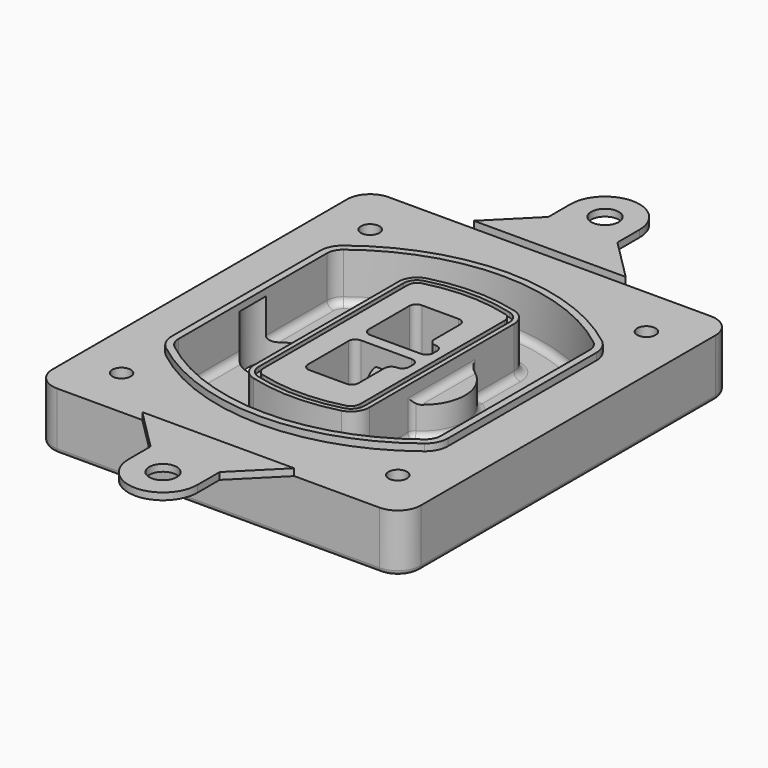
from build123d import *

# Parameters (mm, degrees)
F0_R      = 4
F1_DEPTH  = 25
F2_DEPTH  = 3
F3_DEPTH  = 18
F5_DEPTH  = 21
F6_DEPTH  = 2
F8_DEPTH  = 20
F9_DEPTH  = 16
F10_DEPTH = 25
F7_R      = 6
F7_R_2    = 4
F11_DEPTH = 6
F13_DEPTH = 9
F14_R     = 3
F15_R     = 2
F16_R     = 6
F17_DEPTH = 3


with BuildPart() as f1:
    # F0 (on Top) → F1 (new body)
    with BuildSketch(Plane.XY):
        with BuildLine():
            ThreePointArc((-80, -80), (-77.0710678119, -87.0710678119), (-70, -90))
            Line((-70, -90), (70, -90))
            ThreePointArc((70, -90), (77.0710678119, -87.0710678119), (80, -80))
            Line((80, -80), (80, 80))
            ThreePointArc((80, 80), (77.0710678119, 87.0710678119), (70, 90))
            Line((70, 90), (-70, 90))
            ThreePointArc((-70, 90), (-77.0710678119, 87.0710678119), (-80, 80))
            Line((-80, 80), (-80, -80))
        make_face()
        with Locations((-60, -67.5)):
            Circle(F0_R, mode=Mode.SUBTRACT)
        with Locations((60, -67.5)):
            Circle(F0_R, mode=Mode.SUBTRACT)
        with Locations((-60, 67.5)):
            Circle(F0_R, mode=Mode.SUBTRACT)
        with BuildLine():
            ThreePointArc((-64, 40.2934422872), (-62.5820384798, 46.4328484224), (-58.6153846154, 51.3286200352))
            ThreePointArc((-58.6153846154, 51.3286200352), (0, 71.5), (58.6153846154, 51.3286200352))
            ThreePointArc((58.6153846154, 51.3286200352), (62.5820384798, 46.4328484224), (64, 40.2934422872))
            Line((64, 40.2934422872), (64, -40.2934422872))
            ThreePointArc((64, -40.2934422872), (62.5820384798, -46.4328484224), (58.6153846154, -51.3286200352))
            ThreePointArc((58.6153846154, -51.3286200352), (0, -71.5), (-58.6153846154, -51.3286200352))
            ThreePointArc((-58.6153846154, -51.3286200352), (-62.5820384798, -46.4328484224), (-64, -40.2934422872))
            Line((-64, -40.2934422872), (-64, 40.2934422872))
        make_face(mode=Mode.SUBTRACT)
        with Locations((60, 67.5)):
            Circle(F0_R, mode=Mode.SUBTRACT)
        with BuildLine():
            ThreePointArc((58.6153846154, 51.3286200352), (0, 71.5), (-58.6153846154, 51.3286200352))
            ThreePointArc((-58.6153846154, 51.3286200352), (-62.5820384798, 46.4328484224), (-64, 40.2934422872))
            Line((-64, 40.2934422872), (-64, -40.2934422872))
            ThreePointArc((-64, -40.2934422872), (-62.5820384798, -46.4328484224), (-58.6153846154, -51.3286200352))
            ThreePointArc((-58.6153846154, -51.3286200352), (0, -71.5), (58.6153846154, -51.3286200352))
            ThreePointArc((58.6153846154, -51.3286200352), (62.5820384798, -46.4328484224), (64, -40.2934422872))
            Line((64, -40.2934422872), (64, 40.2934422872))
            ThreePointArc((64, 40.2934422872), (62.5820384798, 46.4328484224), (58.6153846154, 51.3286200352))
        make_face()
        with BuildLine():
            Line((-60, -40.2934422872), (-60, 40.2934422872))
            ThreePointArc((-60, 40.2934422872), (-58.9871703427, 44.6787323838), (-56.1538461538, 48.1757121072))
            ThreePointArc((-56.1538461538, 48.1757121072), (0, 67.5), (56.1538461538, 48.1757121072))
            ThreePointArc((56.1538461538, 48.1757121072), (58.9871703427, 44.6787323838), (60, 40.2934422872))
            Line((60, 40.2934422872), (60, -40.2934422872))
            ThreePointArc((60, -40.2934422872), (58.9871703427, -44.6787323838), (56.1538461538, -48.1757121072))
            ThreePointArc((56.1538461538, -48.1757121072), (0, -67.5), (-56.1538461538, -48.1757121072))
            ThreePointArc((-56.1538461538, -48.1757121072), (-58.9871703427, -44.6787323838), (-60, -40.2934422872))
        make_face(mode=Mode.SUBTRACT)
        with BuildLine():
            ThreePointArc((-56.1538461538, 48.1757121072), (-58.9871703427, 44.6787323838), (-60, 40.2934422872))
            Line((-60, 40.2934422872), (-60, -40.2934422872))
            ThreePointArc((-60, -40.2934422872), (-58.9871703427, -44.6787323838), (-56.1538461538, -48.1757121072))
            ThreePointArc((-56.1538461538, -48.1757121072), (0, -67.5), (56.1538461538, -48.1757121072))
            ThreePointArc((56.1538461538, -48.1757121072), (58.9871703427, -44.6787323838), (60, -40.2934422872))
            Line((60, -40.2934422872), (60, 40.2934422872))
            ThreePointArc((60, 40.2934422872), (58.9871703427, 44.6787323838), (56.1538461538, 48.1757121072))
            ThreePointArc((56.1538461538, 48.1757121072), (0, 67.5), (-56.1538461538, 48.1757121072))
        make_face()
        with BuildLine():
            ThreePointArc((54.3076923077, 45.8110311612), (56.2910192399, 43.3631453548), (57, 40.2934422872))
            Line((57, 40.2934422872), (57, -40.2934422872))
            ThreePointArc((57, -40.2934422872), (56.2910192399, -43.3631453548), (54.3076923077, -45.8110311612))
            ThreePointArc((54.3076923077, -45.8110311612), (0, -64.5), (-54.3076923077, -45.8110311612))
            ThreePointArc((-54.3076923077, -45.8110311612), (-56.2910192399, -43.3631453548), (-57, -40.2934422872))
            Line((-57, -40.2934422872), (-57, 40.2934422872))
            ThreePointArc((-57, 40.2934422872), (-56.2910192399, 43.3631453548), (-54.3076923077, 45.8110311612))
            ThreePointArc((-54.3076923077, 45.8110311612), (0, 64.5), (54.3076923077, 45.8110311612))
        make_face(mode=Mode.SUBTRACT)
        with BuildLine():
            Line((57, -40.2934422872), (57, 40.2934422872))
            ThreePointArc((57, 40.2934422872), (56.2910192399, 43.3631453548), (54.3076923077, 45.8110311612))
            ThreePointArc((54.3076923077, 45.8110311612), (0, 64.5), (-54.3076923077, 45.8110311612))
            ThreePointArc((-54.3076923077, 45.8110311612), (-56.2910192399, 43.3631453548), (-57, 40.2934422872))
            Line((-57, 40.2934422872), (-57, -40.2934422872))
            ThreePointArc((-57, -40.2934422872), (-56.2910192399, -43.3631453548), (-54.3076923077, -45.8110311612))
            ThreePointArc((-54.3076923077, -45.8110311612), (0, -64.5), (54.3076923077, -45.8110311612))
            ThreePointArc((54.3076923077, -45.8110311612), (56.2910192399, -43.3631453548), (57, -40.2934422872))
        make_face()
    extrude(amount=-F1_DEPTH)

    # F0 (on Top) → F2 (join)
    with BuildSketch(Plane.XY):
        with BuildLine():
            ThreePointArc((-56.1538461538, 48.1757121072), (-58.9871703427, 44.6787323838), (-60, 40.2934422872))
            Line((-60, 40.2934422872), (-60, -40.2934422872))
            ThreePointArc((-60, -40.2934422872), (-58.9871703427, -44.6787323838), (-56.1538461538, -48.1757121072))
            ThreePointArc((-56.1538461538, -48.1757121072), (0, -67.5), (56.1538461538, -48.1757121072))
            ThreePointArc((56.1538461538, -48.1757121072), (58.9871703427, -44.6787323838), (60, -40.2934422872))
            Line((60, -40.2934422872), (60, 40.2934422872))
            ThreePointArc((60, 40.2934422872), (58.9871703427, 44.6787323838), (56.1538461538, 48.1757121072))
            ThreePointArc((56.1538461538, 48.1757121072), (0, 67.5), (-56.1538461538, 48.1757121072))
        make_face()
        with BuildLine():
            ThreePointArc((54.3076923077, 45.8110311612), (56.2910192399, 43.3631453548), (57, 40.2934422872))
            Line((57, 40.2934422872), (57, -40.2934422872))
            ThreePointArc((57, -40.2934422872), (56.2910192399, -43.3631453548), (54.3076923077, -45.8110311612))
            ThreePointArc((54.3076923077, -45.8110311612), (0, -64.5), (-54.3076923077, -45.8110311612))
            ThreePointArc((-54.3076923077, -45.8110311612), (-56.2910192399, -43.3631453548), (-57, -40.2934422872))
            Line((-57, -40.2934422872), (-57, 40.2934422872))
            ThreePointArc((-57, 40.2934422872), (-56.2910192399, 43.3631453548), (-54.3076923077, 45.8110311612))
            ThreePointArc((-54.3076923077, 45.8110311612), (0, 64.5), (54.3076923077, 45.8110311612))
        make_face(mode=Mode.SUBTRACT)
    extrude(amount=F2_DEPTH)

    # F0 (on Top) → F3 (cut)
    with BuildSketch(Plane.XY):
        with BuildLine():
            Line((57, -40.2934422872), (57, 40.2934422872))
            ThreePointArc((57, 40.2934422872), (56.2910192399, 43.3631453548), (54.3076923077, 45.8110311612))
            ThreePointArc((54.3076923077, 45.8110311612), (0, 64.5), (-54.3076923077, 45.8110311612))
            ThreePointArc((-54.3076923077, 45.8110311612), (-56.2910192399, 43.3631453548), (-57, 40.2934422872))
            Line((-57, 40.2934422872), (-57, -40.2934422872))
            ThreePointArc((-57, -40.2934422872), (-56.2910192399, -43.3631453548), (-54.3076923077, -45.8110311612))
            ThreePointArc((-54.3076923077, -45.8110311612), (0, -64.5), (54.3076923077, -45.8110311612))
            ThreePointArc((54.3076923077, -45.8110311612), (56.2910192399, -43.3631453548), (57, -40.2934422872))
        make_face()
    extrude(amount=-F3_DEPTH, mode=Mode.SUBTRACT)

    # F4 (on face) → F5 (join, through all)
    with BuildSketch(Plane.XY.offset(3)):
        with BuildLine():
            ThreePointArc((-25, -39.2465276821), (-23.3511545998, -44.1109737193), (-19.0842911877, -46.9702398883))
            ThreePointArc((-19.0842911877, -46.9702398883), (0, -49.5), (19.0842911877, -46.9702398883))
            ThreePointArc((19.0842911877, -46.9702398883), (23.3511545998, -44.1109737193), (25, -39.2465276821))
            Line((25, -39.2465276821), (25, 39.2465276821))
            ThreePointArc((25, 39.2465276821), (23.3511545998, 44.1109737193), (19.0842911877, 46.9702398883))
            ThreePointArc((19.0842911877, 46.9702398883), (0, 49.5), (-19.0842911877, 46.9702398883))
            ThreePointArc((-19.0842911877, 46.9702398883), (-23.3511545998, 44.1109737193), (-25, 39.2465276821))
            Line((-25, 39.2465276821), (-25, -39.2465276821))
        make_face()
        with BuildLine():
            ThreePointArc((18.5632183908, 45.0393118368), (21.7633659499, 42.89486221), (23, 39.2465276821))
            Line((23, 39.2465276821), (23, -39.2465276821))
            ThreePointArc((23, -39.2465276821), (21.7633659499, -42.89486221), (18.5632183908, -45.0393118368))
            ThreePointArc((18.5632183908, -45.0393118368), (0, -47.5), (-18.5632183908, -45.0393118368))
            ThreePointArc((-18.5632183908, -45.0393118368), (-21.7633659499, -42.89486221), (-23, -39.2465276821))
            Line((-23, -39.2465276821), (-23, 39.2465276821))
            ThreePointArc((-23, 39.2465276821), (-21.7633659499, 42.89486221), (-18.5632183908, 45.0393118368))
            ThreePointArc((-18.5632183908, 45.0393118368), (0, 47.5), (18.5632183908, 45.0393118368))
        make_face(mode=Mode.SUBTRACT)
        with BuildLine():
            Line((23, -39.2465276821), (23, 39.2465276821))
            ThreePointArc((23, 39.2465276821), (21.7633659499, 42.89486221), (18.5632183908, 45.0393118368))
            ThreePointArc((18.5632183908, 45.0393118368), (0, 47.5), (-18.5632183908, 45.0393118368))
            ThreePointArc((-18.5632183908, 45.0393118368), (-21.7633659499, 42.89486221), (-23, 39.2465276821))
            Line((-23, 39.2465276821), (-23, -39.2465276821))
            ThreePointArc((-23, -39.2465276821), (-21.7633659499, -42.89486221), (-18.5632183908, -45.0393118368))
            ThreePointArc((-18.5632183908, -45.0393118368), (0, -47.5), (18.5632183908, -45.0393118368))
            ThreePointArc((18.5632183908, -45.0393118368), (21.7633659499, -42.89486221), (23, -39.2465276821))
        make_face()
        with BuildLine():
            ThreePointArc((18.0421455939, 43.1083837852), (20.1755772999, 41.6787507007), (21, 39.2465276821))
            Line((21, 39.2465276821), (21, -39.2465276821))
            ThreePointArc((21, -39.2465276821), (20.1755772999, -41.6787507007), (18.0421455939, -43.1083837852))
            ThreePointArc((18.0421455939, -43.1083837852), (0, -45.5), (-18.0421455939, -43.1083837852))
            ThreePointArc((-18.0421455939, -43.1083837852), (-20.1755772999, -41.6787507007), (-21, -39.2465276821))
            Line((-21, -39.2465276821), (-21, 39.2465276821))
            ThreePointArc((-21, 39.2465276821), (-20.1755772999, 41.6787507007), (-18.0421455939, 43.1083837852))
            ThreePointArc((-18.0421455939, 43.1083837852), (0, 45.5), (18.0421455939, 43.1083837852))
        make_face(mode=Mode.SUBTRACT)
        with BuildLine():
            Line((21, -39.2465276821), (21, 39.2465276821))
            ThreePointArc((21, 39.2465276821), (20.1755772999, 41.6787507007), (18.0421455939, 43.1083837852))
            ThreePointArc((18.0421455939, 43.1083837852), (0, 45.5), (-18.0421455939, 43.1083837852))
            ThreePointArc((-18.0421455939, 43.1083837852), (-20.1755772999, 41.6787507007), (-21, 39.2465276821))
            Line((-21, 39.2465276821), (-21, -39.2465276821))
            ThreePointArc((-21, -39.2465276821), (-20.1755772999, -41.6787507007), (-18.0421455939, -43.1083837852))
            ThreePointArc((-18.0421455939, -43.1083837852), (0, -45.5), (18.0421455939, -43.1083837852))
            ThreePointArc((18.0421455939, -43.1083837852), (20.1755772999, -41.6787507007), (21, -39.2465276821))
        make_face()
        with BuildLine():
            Line((-8, -2.5), (14, -2.5))
            ThreePointArc((14, -2.5), (16.1213203436, -3.3786796564), (17, -5.5))
            Line((17, -5.5), (17, -7.5))
            ThreePointArc((17, -7.5), (16.1213203436, -9.6213203436), (14, -10.5))
            ThreePointArc((14, -10.5), (11.8786796564, -11.3786796564), (11, -13.5))
            Line((11, -13.5), (11, -27.5))
            ThreePointArc((11, -27.5), (10.1213203436, -29.6213203436), (8, -30.5))
            Line((8, -30.5), (-8, -30.5))
            ThreePointArc((-8, -30.5), (-10.1213203436, -29.6213203436), (-11, -27.5))
            Line((-11, -27.5), (-11, -5.5))
            ThreePointArc((-11, -5.5), (-10.1213203436, -3.3786796564), (-8, -2.5))
        make_face(mode=Mode.SUBTRACT)
        with BuildLine():
            ThreePointArc((-8, 2.5), (-10.1213203436, 3.3786796564), (-11, 5.5))
            Line((-11, 5.5), (-11, 27.5))
            ThreePointArc((-11, 27.5), (-10.1213203436, 29.6213203436), (-8, 30.5))
            Line((-8, 30.5), (8, 30.5))
            ThreePointArc((8, 30.5), (10.1213203436, 29.6213203436), (11, 27.5))
            Line((11, 27.5), (11, 13.5))
            ThreePointArc((11, 13.5), (11.8786796564, 11.3786796564), (14, 10.5))
            ThreePointArc((14, 10.5), (16.1213203436, 9.6213203436), (17, 7.5))
            Line((17, 7.5), (17, 5.5))
            ThreePointArc((17, 5.5), (16.1213203436, 3.3786796564), (14, 2.5))
            Line((14, 2.5), (-8, 2.5))
        make_face(mode=Mode.SUBTRACT)
    extrude(amount=-F5_DEPTH)

    # F4 (on face) → F6 (cut)
    with BuildSketch(Plane.XY.offset(3)):
        with BuildLine():
            Line((23, -39.2465276821), (23, 39.2465276821))
            ThreePointArc((23, 39.2465276821), (21.7633659499, 42.89486221), (18.5632183908, 45.0393118368))
            ThreePointArc((18.5632183908, 45.0393118368), (0, 47.5), (-18.5632183908, 45.0393118368))
            ThreePointArc((-18.5632183908, 45.0393118368), (-21.7633659499, 42.89486221), (-23, 39.2465276821))
            Line((-23, 39.2465276821), (-23, -39.2465276821))
            ThreePointArc((-23, -39.2465276821), (-21.7633659499, -42.89486221), (-18.5632183908, -45.0393118368))
            ThreePointArc((-18.5632183908, -45.0393118368), (0, -47.5), (18.5632183908, -45.0393118368))
            ThreePointArc((18.5632183908, -45.0393118368), (21.7633659499, -42.89486221), (23, -39.2465276821))
        make_face()
        with BuildLine():
            ThreePointArc((18.0421455939, 43.1083837852), (20.1755772999, 41.6787507007), (21, 39.2465276821))
            Line((21, 39.2465276821), (21, -39.2465276821))
            ThreePointArc((21, -39.2465276821), (20.1755772999, -41.6787507007), (18.0421455939, -43.1083837852))
            ThreePointArc((18.0421455939, -43.1083837852), (0, -45.5), (-18.0421455939, -43.1083837852))
            ThreePointArc((-18.0421455939, -43.1083837852), (-20.1755772999, -41.6787507007), (-21, -39.2465276821))
            Line((-21, -39.2465276821), (-21, 39.2465276821))
            ThreePointArc((-21, 39.2465276821), (-20.1755772999, 41.6787507007), (-18.0421455939, 43.1083837852))
            ThreePointArc((-18.0421455939, 43.1083837852), (0, 45.5), (18.0421455939, 43.1083837852))
        make_face(mode=Mode.SUBTRACT)
    extrude(amount=-F6_DEPTH, mode=Mode.SUBTRACT)

    # F7 (on face) → F8 (join)
    with BuildSketch(Plane(origin=(0, 0, -25), x_dir=(1, 0, 0), z_dir=(0, 0, -1))):
        with BuildLine():
            ThreePointArc((3.28842436, 0), (16.7567035675, 13.4682792075), (30.224982775, 0))
            Line((30.224982775, 0), (35.224982775, 0))
            ThreePointArc((35.224982775, 0), (16.7567035675, 18.4682792075), (-1.71157564, 0))
            Line((-1.71157564, 0), (3.28842436, 0))
        make_face()
        with BuildLine():
            Line((3.28842436, 0), (30.224982775, 0))
            ThreePointArc((30.224982775, 0), (16.7567035675, 13.4682792075), (3.28842436, 0))
        make_face()
        with BuildLine():
            ThreePointArc((3.28842436, 0), (16.7567035675, -13.4682792075), (30.224982775, 0))
            Line((30.224982775, 0), (3.28842436, 0))
        make_face()
        with BuildLine():
            Line((35.224982775, 0), (30.224982775, 0))
            ThreePointArc((30.224982775, 0), (16.7567035675, -13.4682792075), (3.28842436, 0))
            Line((3.28842436, 0), (-1.71157564, 0))
            ThreePointArc((-1.71157564, 0), (16.7567035675, -18.4682792075), (35.224982775, 0))
        make_face()
    extrude(amount=-F8_DEPTH)

    # F7 (on face) → F9 (cut)
    with BuildSketch(Plane(origin=(0, 0, -25), x_dir=(1, 0, 0), z_dir=(0, 0, -1))):
        with BuildLine():
            Line((3.28842436, 0), (30.224982775, 0))
            ThreePointArc((30.224982775, 0), (16.7567035675, 13.4682792075), (3.28842436, 0))
        make_face()
        with BuildLine():
            ThreePointArc((3.28842436, 0), (16.7567035675, -13.4682792075), (30.224982775, 0))
            Line((30.224982775, 0), (3.28842436, 0))
        make_face()
    extrude(amount=-F9_DEPTH, mode=Mode.SUBTRACT)

    # F7 (on face) → F10 (cut)
    with BuildSketch(Plane(origin=(0, 0, -25), x_dir=(1, 0, 0), z_dir=(0, 0, -1))):
        with BuildLine():
            Line((-59.0318229325, 0), (-32.0952645175, 0))
            ThreePointArc((-32.0952645175, 0), (-45.563543725, 13.4682792075), (-59.0318229325, 0))
        make_face()
        with BuildLine():
            ThreePointArc((-59.0318229325, 0), (-45.563543725, -13.4682792075), (-32.0952645175, 0))
            Line((-32.0952645175, 0), (-59.0318229325, 0))
        make_face()
    extrude(amount=-F10_DEPTH, mode=Mode.SUBTRACT)

    # F7 (on face) → F11 (cut)
    with BuildSketch(Plane(origin=(0, 0, -25), x_dir=(1, 0, 0), z_dir=(0, 0, -1))):
        with Locations((60, -67.5)):
            Circle(F7_R)
        with Locations((60, -67.5)):
            Circle(F7_R_2, mode=Mode.SUBTRACT)
        with Locations((-60, -67.5)):
            Circle(F7_R)
        with Locations((-60, -67.5)):
            Circle(F7_R_2, mode=Mode.SUBTRACT)
        with Locations((-60, 67.5)):
            Circle(F7_R)
        with Locations((-60, 67.5)):
            Circle(F7_R_2, mode=Mode.SUBTRACT)
        with Locations((60, 67.5)):
            Circle(F7_R)
        with Locations((60, 67.5)):
            Circle(F7_R_2, mode=Mode.SUBTRACT)
    extrude(amount=-F11_DEPTH, mode=Mode.SUBTRACT)

    # F12 (on face) → F13 (cut, through all)
    with BuildSketch(Plane(origin=(0, 0, -9), x_dir=(1, 0, 0), z_dir=(0, 0, -1))):
        with BuildLine():
            Line((11, 13.5), (11, 17.5481537753))
            ThreePointArc((11, 17.5481537753), (2.5696536419, 11.8239143813), (-1.5415842455, 2.5))
            Line((-1.5415842455, 2.5), (3.5224848595, 2.5))
            ThreePointArc((3.5224848595, 2.5), (6.1857188154, 8.3455872281), (11.2536447004, 12.2927168648))
            ThreePointArc((11.2536447004, 12.2927168648), (11.0640958889, 12.8831798879), (11, 13.5))
        make_face()
        with BuildLine():
            ThreePointArc((11.2536447004, -12.2927168648), (6.1857188154, -8.3455872281), (3.5224848595, -2.5))
            Line((3.5224848595, -2.5), (-1.5415842455, -2.5))
            ThreePointArc((-1.5415842455, -2.5), (2.5696536419, -11.8239143813), (11, -17.5481537753))
            Line((11, -17.5481537753), (11, -13.5))
            ThreePointArc((11, -13.5), (11.0640958889, -12.8831798879), (11.2536447004, -12.2927168648))
        make_face()
        with BuildLine():
            ThreePointArc((11.2536447004, 12.2927168648), (6.1857188154, 8.3455872281), (3.5224848595, 2.5))
            Line((3.5224848595, 2.5), (14, 2.5))
            ThreePointArc((14, 2.5), (16.1213203436, 3.3786796564), (17, 5.5))
            Line((17, 5.5), (17, 7.5))
            ThreePointArc((17, 7.5), (16.1213203436, 9.6213203436), (14, 10.5))
            ThreePointArc((14, 10.5), (12.3601599782, 10.9878446101), (11.2536447004, 12.2927168648))
        make_face()
        with BuildLine():
            Line((14, -2.5), (3.5224848595, -2.5))
            ThreePointArc((3.5224848595, -2.5), (6.1857188154, -8.3455872281), (11.2536447004, -12.2927168648))
            ThreePointArc((11.2536447004, -12.2927168648), (12.3601599782, -10.9878446101), (14, -10.5))
            ThreePointArc((14, -10.5), (16.1213203436, -9.6213203436), (17, -7.5))
            Line((17, -7.5), (17, -5.5))
            ThreePointArc((17, -5.5), (16.1213203436, -3.3786796564), (14, -2.5))
        make_face()
    extrude(amount=F13_DEPTH, mode=Mode.SUBTRACT)

    # F14
    f14_edges = [f1.edges().sort_by_distance(p)[0] for p in [
        (-57, -23.703476, -18),
        (-57, 23.703476, -18),
        (25, 0, -5),
        (25, 16.526506, -11.5),
        (25, -16.526506, -11.5),
        (25, -27.886517, -18),
        (35.224983, 0, -18),
    ]]
    fillet(f14_edges, radius=F14_R)

    # F15
    f15_edges = [f1.edges().sort_by_distance(p)[0] for p in [
        (0, -90, -25),
    ]]
    fillet(f15_edges, radius=F15_R)


with BuildPart() as f17:
    # F16 (on face) → F17 (new body, through all)
    with BuildSketch(Plane.XY):
        with BuildLine():
            Line((-15, 108), (-33, 90))
            Line((-33, 90), (33, 90))
            Line((33, 90), (15, 108))
            Line((15, 108), (15, 120))
            ThreePointArc((15, 120), (0, 135), (-15, 120))
            Line((-15, 120), (-15, 108))
        make_face()
        with Locations((0, 120)):
            Circle(F16_R, mode=Mode.SUBTRACT)
    extrude(amount=F17_DEPTH)


with BuildPart() as f17b:
    # F16 (on face) → F17, piece 2 (new body, through all)
    with BuildSketch(Plane.XY):
        with BuildLine():
            Line((33, -90), (-33, -90))
            Line((-33, -90), (-15, -108))
            Line((-15, -108), (-15, -120))
            ThreePointArc((-15, -120), (0, -135), (15, -120))
            Line((15, -120), (15, -108))
            Line((15, -108), (33, -90))
        make_face()
        with Locations((0, -120)):
            Circle(F16_R, mode=Mode.SUBTRACT)
    extrude(amount=F17_DEPTH)


solid = Compound([f1.part, f17.part, f17b.part])
